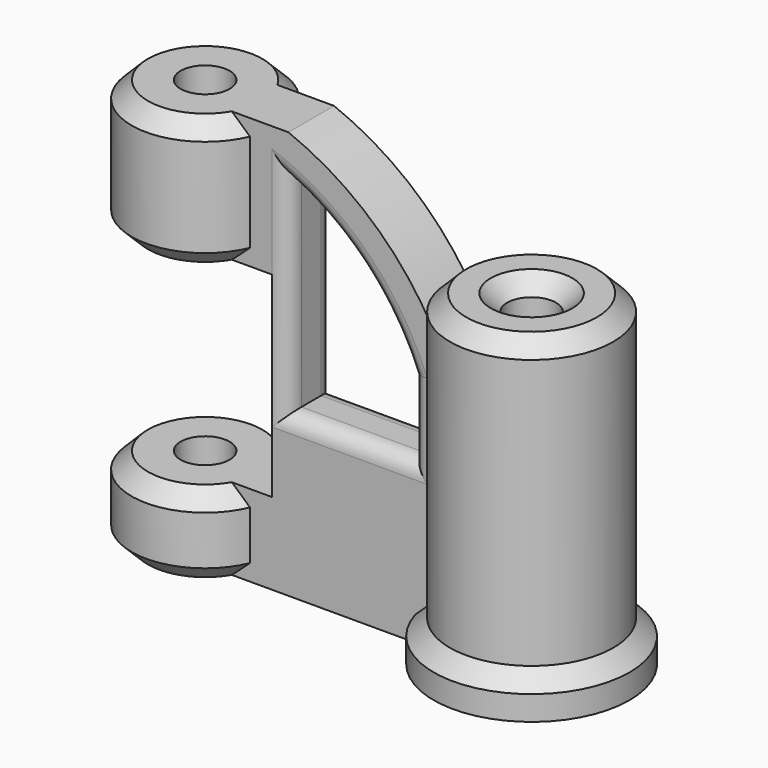
from build123d import *

# Parameters (mm, degrees)
F0_R      = 22.86
F0_R_2    = 7.62
F1_DEPTH  = 127
F0_R_3    = 25.4
F2_DEPTH  = 101.6
F4_DEPTH  = 8.89
F5_W      = 60.96
F5_H      = 60.96
F6_DEPTH  = 50.8
F7_R      = 5.07999
F8_SIZE   = 5.08
F9_R      = 30.48
F10_DEPTH = 12.7
F11_SIZE  = 5.07999


# Not quite as in the source:
# - a fillet or chamfer is up to 0.001 mm smaller than in the source, because OpenCascade refuses the exact size


with BuildPart() as f1:
    # F0 (on Top) → F1 (new body)
    with BuildSketch(Plane.XY):
        with Locations((-101.6, 0)):
            Circle(F0_R)
        with Locations((-101.6, 0)):
            Circle(F0_R_2, mode=Mode.SUBTRACT)
    extrude(amount=F1_DEPTH)



with BuildPart() as f2:
    # F0 (on Top) → F2 (new body)
    with BuildSketch(Plane.XY):
        Circle(F0_R_3)
        Circle(F0_R_2, mode=Mode.SUBTRACT)
    extrude(amount=F2_DEPTH)


with BuildPart() as f1_1:
    add(f1.part)

    add(f2.part)  # F4 merges F2
    # F3 (on Front) → F4 (join, symmetric)
    with BuildSketch(Plane.XZ):
        with BuildLine():
            Line((-81.28, 127), (-81.28, 0))
            Line((-81.28, 0), (-20.32, 0))
            Line((-20.32, 0), (-20.32, 81.28))
            ThreePointArc((-20.32, 81.28), (-40.0155943211, 108.82076155), (-68.58, 127))
            Line((-68.58, 127), (-81.28, 127))
        make_face()
        with BuildLine():
            ThreePointArc((-68.58, 113.1692568198), (-45.7184650999, 96.5627163287), (-30.48, 72.7674195988))
            Line((-30.48, 72.7674195988), (-30.48, 49.6692568198))
            Line((-30.48, 49.6692568198), (-68.58, 49.6692568198))
            Line((-68.58, 49.6692568198), (-68.58, 113.1692568198))
        make_face(mode=Mode.SUBTRACT)
    extrude(amount=F4_DEPTH, both=True)

    # F5 (on Front) → F6 (cut, symmetric)
    with BuildSketch(Plane.XZ):
        with Locations((-104.14, 55.88)):
            Rectangle(F5_W, F5_H)
    extrude(amount=F6_DEPTH, both=True, mode=Mode.SUBTRACT)

    # F7 (radius 5.08 in the source; OpenCascade refuses exactly that, so slightly less here)
    f7_edges = [f1_1.edges().sort_by_distance(p)[0] for p in [
        (-45.718465, -8.89, 96.562716),
        (-30.48, -8.89, 61.218338),
        (-49.53, -8.89, 49.669257),
        (-68.58, -8.89, 81.419257),
        (-45.718465, 8.89, 96.562716),
        (-30.48, 8.89, 61.218338),
        (-49.53, 8.89, 49.669257),
        (-68.58, 8.89, 81.419257),
    ]]
    fillet(f7_edges, radius=F7_R)

    # F8
    f8_edges = [f1_1.edges().sort_by_distance(p)[0] for p in [
        (-124.46, 0, 86.36),
        (-124.46, 0, 0),
        (-124.46, 0, 25.4),
        (-124.46, 0, 127),
    ]]
    chamfer(f8_edges, length=F8_SIZE)

    # F9 (on Top) → F10 (join)
    with BuildSketch(Plane.XY):
        Circle(F9_R)
        with BuildLine():
            Line((-62.23, 2.54), (-62.23, -2.54))
            Line((-62.23, -2.54), (-31.6482369177, -2.54))
            ThreePointArc((-31.6482369177, -2.54), (-31.75, 0), (-31.6482369177, 2.54))
            Line((-31.6482369177, 2.54), (-62.23, 2.54))
        make_face()
    extrude(amount=F10_DEPTH)

    # F11 (size 5.08 in the source; OpenCascade refuses exactly that, so slightly less here)
    f11_edges = [f1_1.edges().sort_by_distance(p)[0] for p in [
        (30.48, 0, 12.7),
        (-25.4, 0, 101.6),
        (-7.62, 0, 101.6),
    ]]
    chamfer(f11_edges, length=F11_SIZE)


solid = f1_1.part
